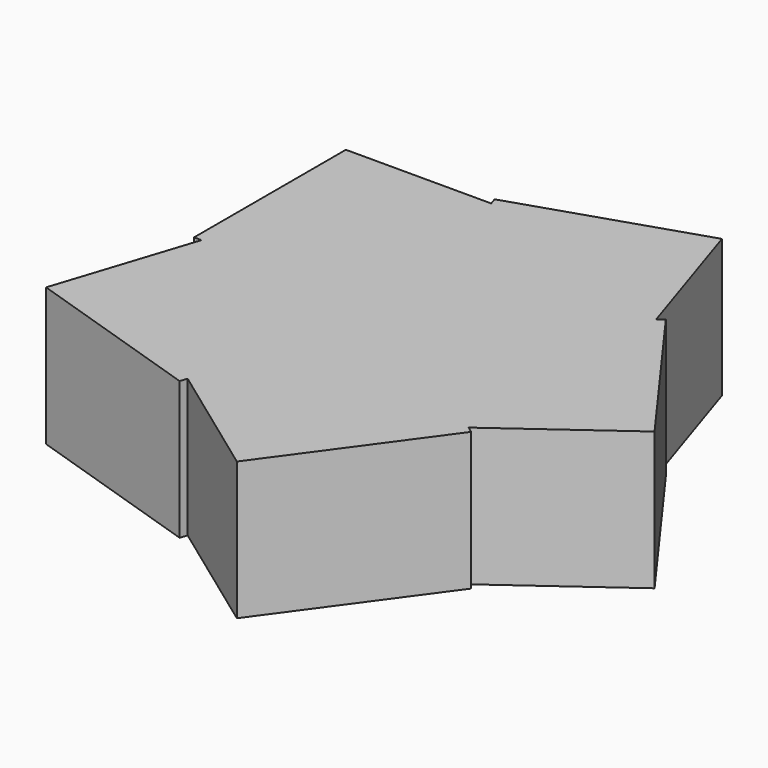
from build123d import *

# Parameters (mm, degrees)
F0_W     = 60
F0_H     = 55
F1_DEPTH = 40
F2_COUNT = 5


with BuildPart() as f1:
    # F0 (on Top) → F1 (new body)
    with BuildSketch(Plane.XY):
        with Locations((-30, 27.5)):
            Rectangle(F0_W, F0_H)
    extrude(amount=F1_DEPTH)

    # F2: F1 ×5 about axis
    f2_axis = Axis((0, 0, 20), (0, 0, -1))


with BuildPart() as f1_1:
    add(f1.part)
    for i in range(1, F2_COUNT):
        add(f1.part.rotate(f2_axis, i * 360 / F2_COUNT))


solid = f1_1.part
